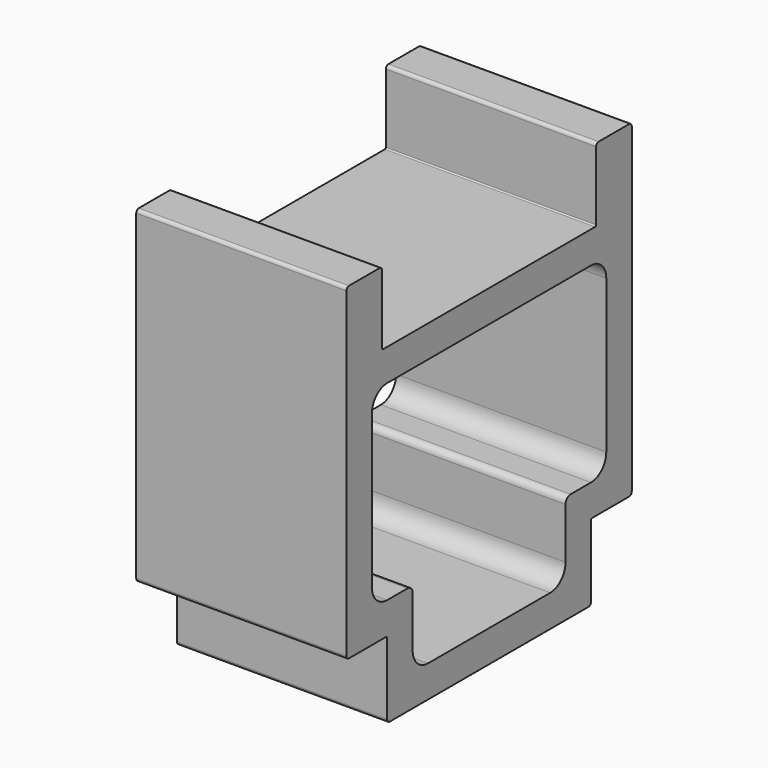
from build123d import *

# Parameters (mm, degrees)
F1_DEPTH    = 33
F2_T        = 5
F2_T3_DEPTH = 43
F3_R        = 0.2
F4_R        = 0.5
F5_R        = 3
F6_R        = 1


# Not quite as in the source:
# - a shell that OpenCascade refuses in one call is made with other operations: the cavity is built on its own and cut out


with BuildPart() as f1:
    # F0 (on Right) → F1 (new body)
    with BuildSketch(Plane.YZ):
        Polygon((-20, 12), (-20, 0), (20, 0), (20, 12), (28, 12), (28, 63.5), (21, 63.5), (21, 52), (-21, 52), (-21, 63.5), (-28, 63.5), (-28, 12), align=None)
    extrude(amount=F1_DEPTH)

    # F2: shell of thickness 5, made by hand


with BuildPart() as f2_core1:
    # F2_t2: copy of F1
    add(f1.part)

    # the walls: a layer under each face that stays
    f2_faces = [f2_core1.faces().sort_by_distance(p)[0] for p in [
        (16.5, -20, 6),
        (16.5, 0, 0),
        (16.5, 20, 6),
        (16.5, 24, 12),
        (16.5, 28, 37.75),
        (16.5, 24.5, 63.5),
        (16.5, 21, 57.75),
        (16.5, 0, 52),
        (16.5, -21, 57.75),
        (16.5, -24.5, 63.5),
        (16.5, -28, 37.75),
        (16.5, -24, 12),
    ]]
    thicken(f2_faces, amount=-F2_T, mode=Mode.SUBTRACT)

    # F2_s4 → F2_t3 (cut)
    with BuildSketch(Plane.YZ.offset(-5)):
        Polygon((-20.05, 11.95), (-15, 12), (-15, 17), (-20, 17), align=None)
        Polygon((20.05, 11.95), (15, 12), (15, 17), (20, 17), align=None)
        Polygon((20.95, 52.05), (26, 52), (26, 47), (21, 47), align=None)
        Polygon((-20.95, 52.05), (-21, 47), (-26, 47), (-26, 52), align=None)
    extrude(amount=F2_T3_DEPTH, mode=Mode.SUBTRACT)


with BuildPart() as f1_1:
    add(f1.part)

    # what is left inside the walls is the cavity
    f2_cavity = [f2_core1.part.solids().sort_by_distance(p)[0] for p in [
        (32.95, 0, 19),
    ]]
    add(f2_cavity, mode=Mode.SUBTRACT)

    # F3
    f3_edges = [f1_1.edges().sort_by_distance(p)[0] for p in [
        (16.5, 20, 12),
        (16.5, -20, 12),
        (16.5, -21, 52),
        (16.5, 21, 52),
    ]]
    fillet(f3_edges, radius=F3_R)

    # F4
    f4_edges = [f1_1.edges().sort_by_distance(p)[0] for p in [
        (16.5, 21, 63.5),
        (16.5, 28, 63.5),
        (16.5, 28, 12),
        (16.5, 20, 0),
        (16.5, -20, 0),
        (16.5, -28, 12),
        (16.5, -28, 63.5),
        (16.5, -21, 63.5),
    ]]
    fillet(f4_edges, radius=F4_R)

    # F5
    f5_edges = [f1_1.edges().sort_by_distance(p)[0] for p in [
        (16.5, -23, 17),
        (16.5, 23, 17),
        (16.5, 15, 5),
        (16.5, -15, 5),
        (16.5, 23, 47),
        (16.5, -23, 47),
    ]]
    fillet(f5_edges, radius=F5_R)

    # F6
    f6_edges = [f1_1.edges().sort_by_distance(p)[0] for p in [
        (16.5, -15, 17),
        (16.5, 15, 17),
    ]]
    fillet(f6_edges, radius=F6_R)


solid = f1_1.part
